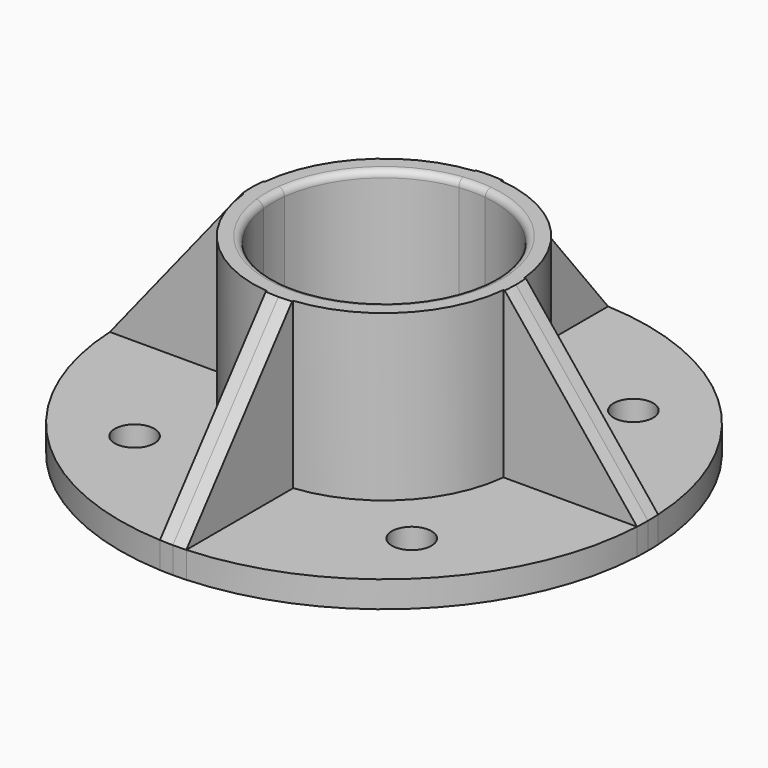
from build123d import *
from build123d import SkipClean  # not in build123d's __all__

# Parameters (mm, degrees)
F1_DEPTH = 25
F0_R     = 3
F2_DEPTH = 4
F3_SIZE2 = 24.99999
F3_SIZE  = 19.99999
F4_R     = 1


# Not quite as in the source:
# - a fillet or chamfer is up to 0.001 mm smaller than in the source, because OpenCascade refuses the exact size


with BuildPart() as f1:
    # F0 (on Top) → F1 (new body)
    with BuildSketch(Plane.XY):
        with BuildLine():
            ThreePointArc((2, 16.6805275696), (11.8793939239, 11.8793939239), (16.6805275696, 2))
            Line((16.6805275696, 2), (19.6987309236, 2))
            ThreePointArc((19.6987309236, 2), (14.0007142675, 14.0007142675), (2, 19.6987309236))
            Line((2, 19.6987309236), (2, 16.6805275696))
        make_face()
        with BuildLine():
            ThreePointArc((-2, 16.6805275696), (0, 16.8), (2, 16.6805275696))
            Line((2, 16.6805275696), (2, 19.6987309236))
            ThreePointArc((2, 19.6987309236), (0, 19.8), (-2, 19.6987309236))
            Line((-2, 19.6987309236), (-2, 16.6805275696))
        make_face()
        with BuildLine():
            ThreePointArc((-16.6805275696, 2), (-11.8793939239, 11.8793939239), (-2, 16.6805275696))
            Line((-2, 16.6805275696), (-2, 19.6987309236))
            ThreePointArc((-2, 19.6987309236), (-14.0007142675, 14.0007142675), (-19.6987309236, 2))
            Line((-19.6987309236, 2), (-16.6805275696, 2))
        make_face()
        with BuildLine():
            ThreePointArc((-16.6805275696, -2), (-16.8, 0), (-16.6805275696, 2))
            Line((-16.6805275696, 2), (-19.6987309236, 2))
            ThreePointArc((-19.6987309236, 2), (-19.8, 0), (-19.6987309236, -2))
            Line((-19.6987309236, -2), (-16.6805275696, -2))
        make_face()
        with BuildLine():
            Line((-2, -19.6987309236), (-2, -16.6805275696))
            ThreePointArc((-2, -16.6805275696), (-11.8793939239, -11.8793939239), (-16.6805275696, -2))
            Line((-16.6805275696, -2), (-19.6987309236, -2))
            ThreePointArc((-19.6987309236, -2), (-14.0007142675, -14.0007142675), (-2, -19.6987309236))
        make_face()
        with BuildLine():
            Line((2, -19.6987309236), (2, -16.6805275696))
            ThreePointArc((2, -16.6805275696), (0, -16.8), (-2, -16.6805275696))
            Line((-2, -16.6805275696), (-2, -19.6987309236))
            ThreePointArc((-2, -19.6987309236), (0, -19.8), (2, -19.6987309236))
        make_face()
        with BuildLine():
            Line((19.6987309236, -2), (16.6805275696, -2))
            ThreePointArc((16.6805275696, -2), (11.8793939239, -11.8793939239), (2, -16.6805275696))
            Line((2, -16.6805275696), (2, -19.6987309236))
            ThreePointArc((2, -19.6987309236), (14.0007142675, -14.0007142675), (19.6987309236, -2))
        make_face()
        with BuildLine():
            ThreePointArc((16.6805275696, 2), (16.7701052944, 1.0017826188), (16.8, 0))
            ThreePointArc((16.8, 0), (16.7701052944, -1.0017826188), (16.6805275696, -2))
            Line((16.6805275696, -2), (19.6987309236, -2))
            ThreePointArc((19.6987309236, -2), (19.7746665242, -1.0012811076), (19.8, 0))
            ThreePointArc((19.8, 0), (19.7746665242, 1.0012811076), (19.6987309236, 2))
            Line((19.6987309236, 2), (16.6805275696, 2))
        make_face()
        with BuildLine():
            ThreePointArc((-19.6987309236, -2), (-19.8, 0), (-19.6987309236, 2))
            Line((-19.6987309236, 2), (-39.9499687109, 2))
            ThreePointArc((-39.9499687109, 2), (-39.9874902215, 1.0003128423), (-40, 0))
            ThreePointArc((-40, 0), (-39.9874902215, -1.0003128423), (-39.9499687109, -2))
            Line((-39.9499687109, -2), (-19.6987309236, -2))
        make_face()
        with BuildLine():
            Line((2, -39.9499687109), (2, -19.6987309236))
            ThreePointArc((2, -19.6987309236), (0, -19.8), (-2, -19.6987309236))
            Line((-2, -19.6987309236), (-2, -39.9499687109))
            ThreePointArc((-2, -39.9499687109), (-1.0003128423, -39.9874902215), (0, -40))
            ThreePointArc((0, -40), (1.0003128423, -39.9874902215), (2, -39.9499687109))
        make_face()
        with BuildLine():
            Line((39.9499687109, 2), (19.6987309236, 2))
            ThreePointArc((19.6987309236, 2), (19.7746665242, 1.0012811076), (19.8, 0))
            ThreePointArc((19.8, 0), (19.7746665242, -1.0012811076), (19.6987309236, -2))
            Line((19.6987309236, -2), (39.9499687109, -2))
            ThreePointArc((39.9499687109, -2), (39.9874902215, -1.0003128423), (40, 0))
            ThreePointArc((40, 0), (39.9874902215, 1.0003128423), (39.9499687109, 2))
        make_face()
        with BuildLine():
            ThreePointArc((-2, 19.6987309236), (0, 19.8), (2, 19.6987309236))
            Line((2, 19.6987309236), (2, 39.9499687109))
            ThreePointArc((2, 39.9499687109), (1.0003128423, 39.9874902215), (0, 40))
            ThreePointArc((0, 40), (-1.0003128423, 39.9874902215), (-2, 39.9499687109))
            Line((-2, 39.9499687109), (-2, 19.6987309236))
        make_face()
    extrude(amount=F1_DEPTH)

    # F0 (on Top) → F2 (join)
    with BuildSketch(Plane.XY):
        with BuildLine():
            ThreePointArc((-19.6987309236, 2), (-14.0007142675, 14.0007142675), (-2, 19.6987309236))
            Line((-2, 19.6987309236), (-2, 39.9499687109))
            ThreePointArc((-2, 39.9499687109), (-28.2842712475, 28.2842712475), (-39.9499687109, 2))
            Line((-39.9499687109, 2), (-19.6987309236, 2))
        make_face()
        with Locations((-21, 21)):
            Circle(F0_R, mode=Mode.SUBTRACT)
        with BuildLine():
            ThreePointArc((2, 19.6987309236), (14.0007142675, 14.0007142675), (19.6987309236, 2))
            Line((19.6987309236, 2), (39.9499687109, 2))
            ThreePointArc((39.9499687109, 2), (28.2842712475, 28.2842712475), (2, 39.9499687109))
            Line((2, 39.9499687109), (2, 19.6987309236))
        make_face()
        with Locations((21, 21)):
            Circle(F0_R, mode=Mode.SUBTRACT)
        with BuildLine():
            Line((39.9499687109, 2), (19.6987309236, 2))
            ThreePointArc((19.6987309236, 2), (19.7746665242, 1.0012811076), (19.8, 0))
            ThreePointArc((19.8, 0), (19.7746665242, -1.0012811076), (19.6987309236, -2))
            Line((19.6987309236, -2), (39.9499687109, -2))
            ThreePointArc((39.9499687109, -2), (39.9874902215, -1.0003128423), (40, 0))
            ThreePointArc((40, 0), (39.9874902215, 1.0003128423), (39.9499687109, 2))
        make_face()
        with BuildLine():
            ThreePointArc((-2, 19.6987309236), (0, 19.8), (2, 19.6987309236))
            Line((2, 19.6987309236), (2, 39.9499687109))
            ThreePointArc((2, 39.9499687109), (1.0003128423, 39.9874902215), (0, 40))
            ThreePointArc((0, 40), (-1.0003128423, 39.9874902215), (-2, 39.9499687109))
            Line((-2, 39.9499687109), (-2, 19.6987309236))
        make_face()
        with BuildLine():
            Line((39.9499687109, -2), (19.6987309236, -2))
            ThreePointArc((19.6987309236, -2), (14.0007142675, -14.0007142675), (2, -19.6987309236))
            Line((2, -19.6987309236), (2, -39.9499687109))
            ThreePointArc((2, -39.9499687109), (28.2842712475, -28.2842712475), (39.9499687109, -2))
        make_face()
        with Locations((21, -21)):
            Circle(F0_R, mode=Mode.SUBTRACT)
        with BuildLine():
            Line((19.6987309236, -2), (16.6805275696, -2))
            ThreePointArc((16.6805275696, -2), (11.8793939239, -11.8793939239), (2, -16.6805275696))
            Line((2, -16.6805275696), (2, -19.6987309236))
            ThreePointArc((2, -19.6987309236), (14.0007142675, -14.0007142675), (19.6987309236, -2))
        make_face()
        with BuildLine():
            ThreePointArc((16.6805275696, 2), (16.7701052944, 1.0017826188), (16.8, 0))
            ThreePointArc((16.8, 0), (16.7701052944, -1.0017826188), (16.6805275696, -2))
            Line((16.6805275696, -2), (19.6987309236, -2))
            ThreePointArc((19.6987309236, -2), (19.7746665242, -1.0012811076), (19.8, 0))
            ThreePointArc((19.8, 0), (19.7746665242, 1.0012811076), (19.6987309236, 2))
            Line((19.6987309236, 2), (16.6805275696, 2))
        make_face()
        with BuildLine():
            ThreePointArc((2, 16.6805275696), (11.8793939239, 11.8793939239), (16.6805275696, 2))
            Line((16.6805275696, 2), (19.6987309236, 2))
            ThreePointArc((19.6987309236, 2), (14.0007142675, 14.0007142675), (2, 19.6987309236))
            Line((2, 19.6987309236), (2, 16.6805275696))
        make_face()
        with BuildLine():
            Line((2, -19.6987309236), (2, -16.6805275696))
            ThreePointArc((2, -16.6805275696), (0, -16.8), (-2, -16.6805275696))
            Line((-2, -16.6805275696), (-2, -19.6987309236))
            ThreePointArc((-2, -19.6987309236), (0, -19.8), (2, -19.6987309236))
        make_face()
        with BuildLine():
            Line((2, -39.9499687109), (2, -19.6987309236))
            ThreePointArc((2, -19.6987309236), (0, -19.8), (-2, -19.6987309236))
            Line((-2, -19.6987309236), (-2, -39.9499687109))
            ThreePointArc((-2, -39.9499687109), (-1.0003128423, -39.9874902215), (0, -40))
            ThreePointArc((0, -40), (1.0003128423, -39.9874902215), (2, -39.9499687109))
        make_face()
        with BuildLine():
            Line((-2, -19.6987309236), (-2, -16.6805275696))
            ThreePointArc((-2, -16.6805275696), (-11.8793939239, -11.8793939239), (-16.6805275696, -2))
            Line((-16.6805275696, -2), (-19.6987309236, -2))
            ThreePointArc((-19.6987309236, -2), (-14.0007142675, -14.0007142675), (-2, -19.6987309236))
        make_face()
        with BuildLine():
            Line((-2, -39.9499687109), (-2, -19.6987309236))
            ThreePointArc((-2, -19.6987309236), (-14.0007142675, -14.0007142675), (-19.6987309236, -2))
            Line((-19.6987309236, -2), (-39.9499687109, -2))
            ThreePointArc((-39.9499687109, -2), (-28.2842712475, -28.2842712475), (-2, -39.9499687109))
        make_face()
        with Locations((-21, -21)):
            Circle(F0_R, mode=Mode.SUBTRACT)
        with BuildLine():
            ThreePointArc((-19.6987309236, -2), (-19.8, 0), (-19.6987309236, 2))
            Line((-19.6987309236, 2), (-39.9499687109, 2))
            ThreePointArc((-39.9499687109, 2), (-39.9874902215, 1.0003128423), (-40, 0))
            ThreePointArc((-40, 0), (-39.9874902215, -1.0003128423), (-39.9499687109, -2))
            Line((-39.9499687109, -2), (-19.6987309236, -2))
        make_face()
        with BuildLine():
            ThreePointArc((-16.6805275696, -2), (-16.8, 0), (-16.6805275696, 2))
            Line((-16.6805275696, 2), (-19.6987309236, 2))
            ThreePointArc((-19.6987309236, 2), (-19.8, 0), (-19.6987309236, -2))
            Line((-19.6987309236, -2), (-16.6805275696, -2))
        make_face()
        with BuildLine():
            ThreePointArc((-16.6805275696, 2), (-11.8793939239, 11.8793939239), (-2, 16.6805275696))
            Line((-2, 16.6805275696), (-2, 19.6987309236))
            ThreePointArc((-2, 19.6987309236), (-14.0007142675, 14.0007142675), (-19.6987309236, 2))
            Line((-19.6987309236, 2), (-16.6805275696, 2))
        make_face()
        with BuildLine():
            ThreePointArc((-2, 16.6805275696), (0, 16.8), (2, 16.6805275696))
            Line((2, 16.6805275696), (2, 19.6987309236))
            ThreePointArc((2, 19.6987309236), (0, 19.8), (-2, 19.6987309236))
            Line((-2, 19.6987309236), (-2, 16.6805275696))
        make_face()
    with SkipClean():  # cleaning this boolean's faces spoils the solid; the shape is the same uncleaned
        extrude(amount=-F2_DEPTH)

    # F3 (size 20 and 25 in the source; OpenCascade refuses exactly that, so slightly less here)
    f3_edges = [f1.edges().sort_by_distance(p)[0] for p in [
        (-40, 0, 25),
        (0, -40, 25),
        (40, 0, 25),
        (0, 40, 25),
    ]]
    f3_side = f1.faces().sort_by_distance((-29.82435, 0.868629, 25))[0]
    chamfer(f3_edges, length=F3_SIZE, length2=F3_SIZE2, reference=f3_side)

    # F4
    f4_edges = [f1.edges().sort_by_distance(p)[0] for p in [
        (-16.680528, -2, 25),
    ]]
    fillet(f4_edges, radius=F4_R)


solid = f1.part
